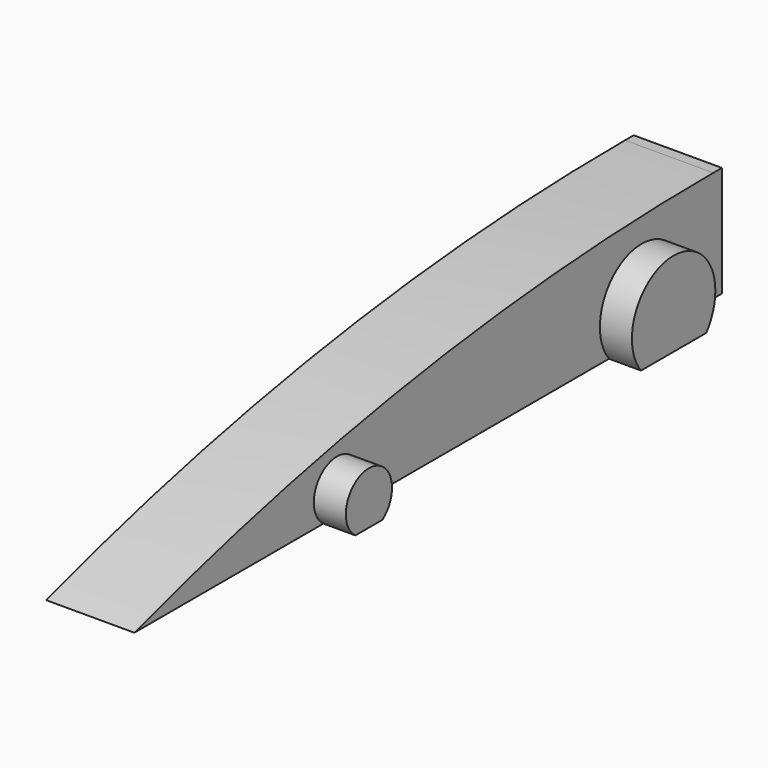
from build123d import *

# Parameters (mm, degrees)
F0_W        = 215.5817523599
F0_H        = 32.4833281338
F1_DEPTH    = 25.908
F2_T1_DEPTH = 1087.9500123763
F4_DEPTH    = 9.398


# Not quite as in the source:
# - a fillet or chamfer that OpenCascade refuses, or shapes differently, is made with other operations: its cross-section is extruded or revolved along the edge and cut away or added


with BuildPart() as f1:
    # F0 (on Right) → F1 (new body)
    with BuildSketch(Plane.YZ):
        with Locations((-13.4214349091, 16.2416640669)):
            Rectangle(F0_W, F0_H)
    extrude(amount=-F1_DEPTH)

    # F2: fillet of radius 710.7106737728 on 1 edges, made by hand

    # F2_s2 → F2_t1 (cut)
    with BuildSketch(Plane.YZ.offset(-556.9290061881)):
        with BuildLine():
            ThreePointArc((91.1960913862, 32.4833281338), (-16.2428401618, 24.3155625185), (-121.212311089, 0))
            Line((-121.212311089, 0), (-121.212311089, 32.4833281338))
            Line((-121.212311089, 32.4833281338), (91.1960913862, 32.4833281338))
        make_face()
    extrude(amount=F2_T1_DEPTH, mode=Mode.SUBTRACT)

    # F3 (on face) → F4 (join)
    with BuildSketch(Plane.YZ):
        with BuildLine():
            ThreePointArc((-41.9370249708, 0), (-39.3490534124, 3.0127715747), (-38.4182262134, 6.873853039))
            ThreePointArc((-38.4182262134, 6.873853039), (-50.7526254785, 14.4163436408), (-51.8460630576, 0))
            Line((-51.8460630576, 0), (-41.9370249708, 0))
        make_face()
        with BuildLine():
            ThreePointArc((80.2152858595, 9.5448940992), (59.8493914636, 23.9956386528), (52.9354202211, 0))
            Line((52.9354202211, 0), (76.8756431877, 0))
            ThreePointArc((76.8756431877, 0), (79.356276258, 4.4887538584), (80.2152858595, 9.5448940992))
        make_face()
    extrude(amount=F4_DEPTH)


solid = f1.part
